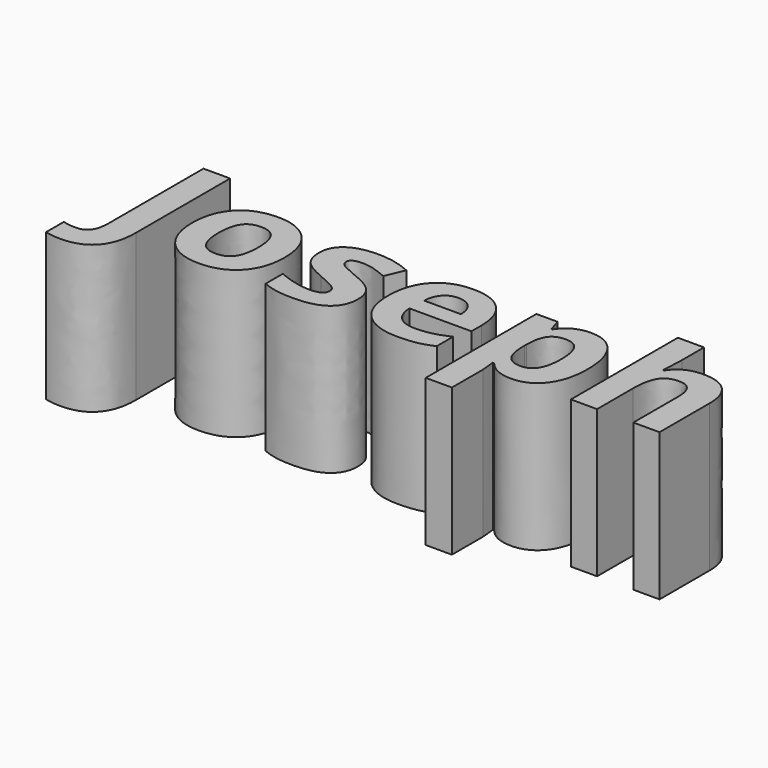
from build123d import *

# Parameters (mm, degrees)
F0_TEXT_SIZE = 30.3620200915
F1_DEPTH     = 25.4


# Not quite as in the source:
# - Text() gives the source's letters only with a copy of the font that has no kerning and outlines rounded to 1/6400 em; it was checked with that copy


with BuildPart() as f1:
    # F0 (on Top) → F1 (new body)
    with BuildSketch(Plane.XY):
        with Locations((-42.555404827, 26.9614765421)):
            Text('Joseph', F0_TEXT_SIZE, font='Open Sans', font_style=FontStyle.BOLD, text_align=(TextAlign.LEFT, TextAlign.BOTTOM))
    extrude(amount=F1_DEPTH)


solid = f1.part
